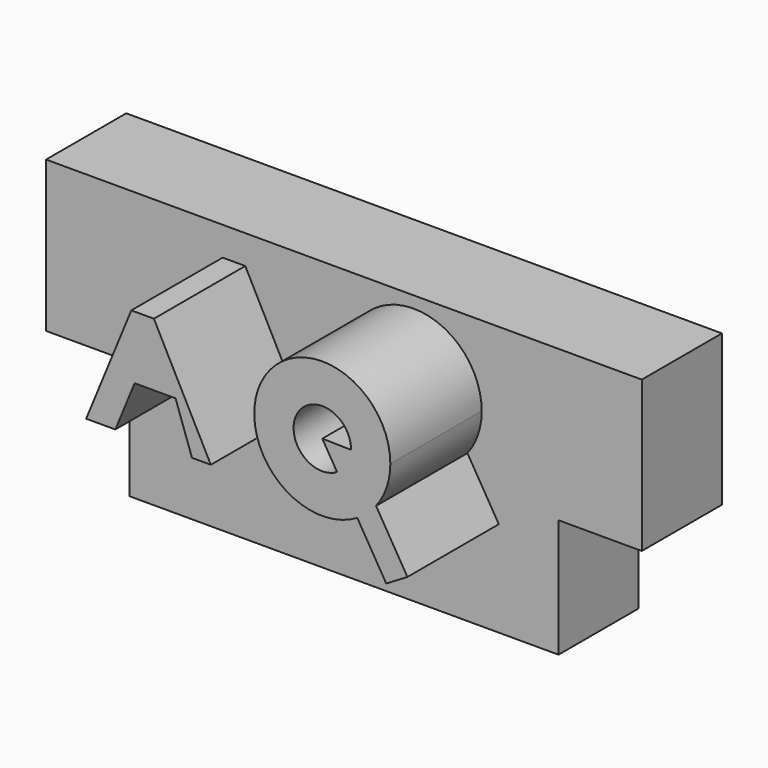
from build123d import *

# Parameters (mm, degrees)
F1_DEPTH = 11.1375302076
F3_DEPTH = 25.4


# Not quite as in the source:
# - a feature names something its author has since deleted; it is built from what else it names


with BuildPart() as f1:
    # F0 (on Front) → F1 (new body, symmetric)
    with BuildSketch(Plane.XZ):
        Polygon((-47.7266, 0), (0, 0), (0, 33.5543528199), (-66.2321434704, 33.5543528199), (-66.2321434704, 0), align=None)
        Polygon((47.7266, 0), (0, 0), (0, -26.3268053532), (23.8633, -26.3268053532), (47.7266, -26.3268053532), align=None)
        Polygon((0, 33.5543528199), (0, 0), (47.7266, 0), (66.2432, 0), (66.2432, 33.5543528199), align=None)
        Polygon((0, -26.3268053532), (0, 0), (-47.7266, 0), (-47.7266, -26.3268053532), (-23.8633, -26.3268053532), align=None)
    extrude(amount=F1_DEPTH, both=True)

    # F2 (on face) → F3 (join)
    with BuildSketch(Plane.XZ.offset(11.1375302076)):
        Polygon((-21.9350446656, 23.558561476), (-26.957899332, 27.1239373833), (-37.0000749826, 2.6461503003), (-30.5145010352, 2.6461503003), (-26.2247728504, 13.1023558882), align=None)
        Polygon((-21.9350446656, 27.1239373833), (-26.957899332, 27.1239373833), (-21.9350446656, 23.558561476), (-17.1249434352, 13.1023558882), (-13.4637281299, 2.6461503003), (-9.2794969678, 2.6461503003), align=None)
        Polygon((-17.1249434352, 13.1023558882), (-21.9350446656, 23.558561476), (-26.2247728504, 13.1023558882), align=None)
        with BuildLine():
            ThreePointArc((21.8997799497, 15.7127540144), (21.0422650014, 12.6276476595), (18.7955158738, 10.3461281077))
            Line((18.7955158738, 10.3461281077), (23.2909736673, 2.8426809347))
            ThreePointArc((23.2909736673, 2.8426809347), (25.5526183138, 4.5004893654), (27.4696294265, 6.5470556834))
            Line((27.4696294265, 6.5470556834), (21.9791319159, 15.7113410392))
            Line((21.9791319159, 15.7113410392), (21.8997799497, 15.7127540144))
        make_face()
        with BuildLine():
            Line((23.2909736673, 2.8426809347), (18.7955158738, 10.3461281077))
            ThreePointArc((18.7955158738, 10.3461281077), (9.9537248959, 18.9759861326), (21.9007925331, 15.8264953643))
            ThreePointArc((21.9007925331, 15.8264953643), (21.9005393822, 15.7696224358), (21.8997799497, 15.7127540144))
            Line((21.8997799497, 15.7127540144), (21.9791319159, 15.7113410392))
            Line((21.9791319159, 15.7113410392), (27.4696294265, 6.5470556834))
            ThreePointArc((27.4696294265, 6.5470556834), (29.8312607656, 10.9221852492), (30.6478411926, 15.8264953643))
            ThreePointArc((30.6478411926, 15.8264953643), (2.3434407909, 23.2881127649), (23.2909736673, 2.8426809347))
        make_face()
        with BuildLine():
            ThreePointArc((27.4696294265, 6.5470556834), (25.5526183138, 4.5004893654), (23.2909736673, 2.8426809347))
            Line((23.2909736673, 2.8426809347), (29.7385305166, -7.9190488905))
            Line((29.7385305166, -7.9190488905), (34.4466119702, -5.0983478214))
            Line((34.4466119702, -5.0983478214), (27.4696294265, 6.5470556834))
        make_face()
        with BuildLine():
            Line((21.8997799497, 15.7127540144), (15.512123704, 15.8264953643))
            Line((15.512123704, 15.8264953643), (18.7955158738, 10.3461281077))
            ThreePointArc((18.7955158738, 10.3461281077), (21.0422650014, 12.6276476595), (21.8997799497, 15.7127540144))
        make_face()
    extrude(amount=F3_DEPTH)


solid = f1.part
